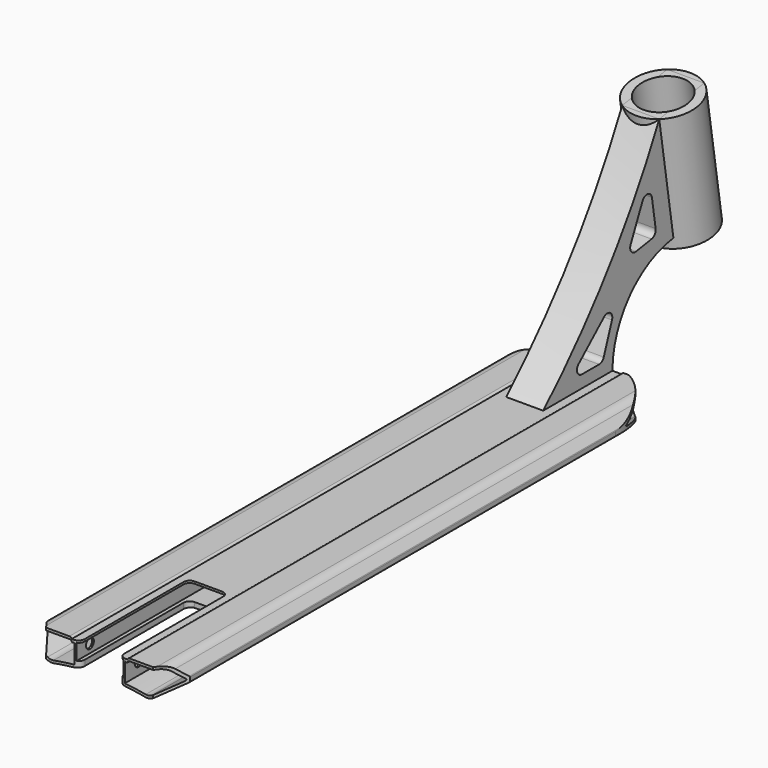
from build123d import *

# Parameters (mm, degrees)
F1_DEPTH       = 250
F2_W           = 38
F2_H           = 13
F3_DEPTH       = 250
F4_T1_DEPTH    = 509.3674969976
F5_R           = 9
F6_R           = 1
F8_DEPTH       = 500.001
F10_DEPTH      = 22.2193051812
F10_DEPTH_BACK = 1.301
F12_DEPTH      = 22.219305294
F12_DEPTH_BACK = 1.3010001
F13_T1_DEPTH   = 1.7268039449
F13_T6_DEPTH   = 34.5366784866
F13_S7_R       = 200
F13_T8_DEPTH   = 19
F13_T12_DEPTH  = 64.5366784866
F13_T18_DEPTH  = 31.7268039449
F13_S19_R      = 200
F13_T20_DEPTH  = 18
F13_T25_DEPTH  = 31.7268039449
F13_S26_R      = 200
F13_T27_DEPTH  = 18
F13_T32_DEPTH  = 64.5366784866
F13_T38_DEPTH  = 34.5366784866
F13_S39_R      = 200
F13_T40_DEPTH  = 19
F13_T41_DEPTH  = 61.7268039449
F15_DEPTH      = 15
F16_R          = 27.5
F17_DEPTH      = 100
F19_D          = 40
F21_D          = 8
F21_DEPTH      = 50
F21_TIP        = 2.4034424761
F23_DEPTH      = 42.5010001
F23_DEPTH_BACK = 72.5010001
F24_R          = 5


# Not quite as in the source:
# - a fillet or chamfer that OpenCascade refuses, or shapes differently, is made with other operations: its cross-section is extruded or revolved along the edge and cut away or added


with BuildPart() as f1:
    # F0 (on Front) → F1 (new body, symmetric)
    with BuildSketch(Plane.XZ):
        with BuildLine():
            Line((22.5, 0), (0, 0))
            Line((0, 0), (-22.5, 0))
            Line((-22.5, 0), (-22.5, 1.3))
            Line((-22.5, 1.3), (-49.1090036882, 1.3))
            Line((-49.1090036882, 1.3), (-57.5, -8.7))
            Line((-57.5, -8.7), (-57.5, -12.7))
            Line((-57.5, -12.7), (-40.1794919243, -22.7))
            ThreePointArc((-40.1794919243, -22.7), (0, -18.6224551416), (40.1794919243, -22.7))
            Line((40.1794919243, -22.7), (57.5, -12.7))
            Line((57.5, -12.7), (57.5, -8.7))
            Line((57.5, -8.7), (49.1090036882, 1.3))
            Line((49.1090036882, 1.3), (22.5, 1.3))
            Line((22.5, 1.3), (22.5, 0))
        make_face()
    extrude(amount=F1_DEPTH, both=True)

    # F2 (on Front) → F3 (cut, symmetric)
    with BuildSketch(Plane.XZ):
        with Locations((0, -8.2268039449)):
            Rectangle(F2_W, F2_H)
    extrude(amount=F3_DEPTH, both=True, mode=Mode.SUBTRACT)

    # F4: fillet of radius 2 on 2 edges, made by hand

    # F4_s2 → F4_t1 (cut)
    with BuildSketch(Plane.XZ.offset(-254.6837484988)):
        with BuildLine():
            ThreePointArc((24.3734993995, 1.3), (23.2333239744, 0.9431676725), (22.5, 0))
            Line((22.5, 0), (22.5, 1.3))
            Line((22.5, 1.3), (24.3734993995, 1.3))
        make_face()
        with BuildLine():
            ThreePointArc((-24.3734993995, 1.3), (-23.2333239744, 0.9431676725), (-22.5, 0))
            Line((-22.5, 0), (-22.5, 1.3))
            Line((-22.5, 1.3), (-24.3734993995, 1.3))
        make_face()
    extrude(amount=F4_T1_DEPTH, mode=Mode.SUBTRACT)

    # F5
    f5_edges = [f1.edges().sort_by_distance(p)[0] for p in [
        (-49.109004, 0, 1.3),
        (49.109004, 0, 1.3),
        (40.179492, 0, -22.7),
        (-40.179492, 0, -22.7),
    ]]
    fillet(f5_edges, radius=F5_R)

    # F6
    f6_edges = [f1.edges().sort_by_distance(p)[0] for p in [
        (-57.5, 0, -8.7),
        (-57.5, 0, -12.7),
        (57.5, 0, -8.7),
        (57.5, 0, -12.7),
    ]]
    fillet(f6_edges, radius=F6_R)

    # F7 (on face) → F8 (cut, through all)
    with BuildSketch(Plane.XZ.offset(250)):
        with BuildLine():
            ThreePointArc((-37.3093701274, -20.0978700124), (-28.8874083403, -18.698675567), (-20.4138456833, -17.6566000706))
            Line((-20.4138456833, -17.6566000706), (-20.4138456833, -2.3003034743))
            Line((-20.4138456833, -2.3003034743), (-22.4138456833, -2.3003034743))
            ThreePointArc((-22.4138456833, -2.3003034743), (-23.1084683824, -1.1509046105), (-24.3734993995, -0.7))
            Line((-24.3734993995, -0.7), (-44.9122347648, -0.7))
            ThreePointArc((-44.9122347648, -0.7), (-47.870562597, -1.3558454907), (-50.2745458667, -3.2004867322))
            Line((-50.2745458667, -3.2004867322), (-55.9308095341, -9.9413592785))
            ThreePointArc((-55.9308095341, -9.9413592785), (-56.149572844, -10.7577950659), (-55.664765091, -11.450172292))
            Line((-55.664765091, -11.450172292), (-42.1022690923, -19.2804830077))
            ThreePointArc((-42.1022690923, -19.2804830077), (-39.7790673433, -20.1186780608), (-37.3093701274, -20.0978700124))
        make_face()
        with BuildLine():
            Line((22.4138456833, -2.3003034743), (20.4138456833, -2.3003034743))
            Line((20.4138456833, -2.3003034743), (20.4138456833, -17.6566000706))
            ThreePointArc((20.4138456833, -17.6566000706), (28.8874083403, -18.698675567), (37.3093701274, -20.0978700124))
            ThreePointArc((37.3093701274, -20.0978700124), (39.7790673433, -20.1186780608), (42.1022690923, -19.2804830077))
            Line((42.1022690923, -19.2804830077), (55.664765091, -11.450172292))
            ThreePointArc((55.664765091, -11.450172292), (56.149572844, -10.7577950659), (55.9308095341, -9.9413592785))
            Line((55.9308095341, -9.9413592785), (50.2745458667, -3.2004867322))
            ThreePointArc((50.2745458667, -3.2004867322), (47.870562597, -1.3558454907), (44.9122347648, -0.7))
            Line((44.9122347648, -0.7), (24.3734993995, -0.7))
            ThreePointArc((24.3734993995, -0.7), (23.1084683824, -1.1509046105), (22.4138456833, -2.3003034743))
        make_face()
    extrude(amount=-F8_DEPTH, mode=Mode.SUBTRACT)

    # F9 (on Top) → F10 (cut, two sides)
    with BuildSketch(Plane.XY) as f10_sk:
        with BuildLine():
            ThreePointArc((-57.5, 200), (0, 257.5), (57.5, 200))
            Line((57.5, 200), (57.5, 280))
            Line((57.5, 280), (-57.5, 280))
            Line((-57.5, 280), (-57.5, 200))
        make_face()
    extrude(amount=-F10_DEPTH, mode=Mode.SUBTRACT)
    extrude(f10_sk.sketch, amount=F10_DEPTH_BACK, mode=Mode.SUBTRACT)

    # F11 (on Top) → F12 (cut, two sides)
    with BuildSketch(Plane.XY) as f12_sk:
        Polygon((16, -140), (-16, -140), (-16, -250), (-43.2975540478, -250), (-68, -216), (-68, -346), (68, -346), (68, -216), (43.2975540478, -250), (16, -250), align=None)
    extrude(amount=-F12_DEPTH, mode=Mode.SUBTRACT)
    extrude(f12_sk.sketch, amount=F12_DEPTH_BACK, mode=Mode.SUBTRACT)

    # F13: fillet of radius 5 on 6 edges, made by hand

    # F13_s2 → F13_t1 (join)
    with BuildSketch(Plane.XY.offset(-1.7268039449)):
        with BuildLine():
            ThreePointArc((-11, -140), (-14.5355339059, -141.4644660941), (-16, -145))
            Line((-16, -145), (-16.1, -145))
            Line((-16.1, -145), (-16.1, -139.9))
            Line((-16.1, -139.9), (-11, -139.9))
            Line((-11, -139.9), (-11, -140))
        make_face()
        with BuildLine():
            ThreePointArc((16, -145), (14.5355339059, -141.4644660941), (11, -140))
            Line((11, -140), (11, -139.9))
            Line((11, -139.9), (16.1, -139.9))
            Line((16.1, -139.9), (16.1, -145))
            Line((16.1, -145), (16, -145))
        make_face()
    extrude(amount=F13_T1_DEPTH)


with BuildPart() as f13_tool4:
    # F13_s5 → F13_t6 (new body)
    with BuildSketch(Plane.XY.offset(-49.2634824315)):
        with BuildLine():
            ThreePointArc((-16, -145), (-14.5355339059, -141.4644660941), (-11, -140))
            Line((-11, -140), (-11, -139.9))
            Line((-11, -139.9), (-16.1, -139.9))
            Line((-16.1, -139.9), (-16.1, -145))
            Line((-16.1, -145), (-16, -145))
        make_face()
    extrude(amount=F13_T6_DEPTH)

    # F13_s7 → F13_t8 (cut, symmetric)
    with BuildSketch(Plane.XZ.offset(142.4)):
        with Locations((0, -218.6224551416)):
            Circle(F13_S7_R)
    extrude(amount=F13_T8_DEPTH, both=True, mode=Mode.SUBTRACT)


with BuildPart() as f1_1:
    add(f1.part)

    # F13_t3: union F13_tool4
    add(f13_tool4.part)


with BuildPart() as f13_tool10:
    # F13_s11 → F13_t12 (new body)
    with BuildSketch(Plane.XY.offset(-49.2634824315)):
        with BuildLine():
            ThreePointArc((-16, -145), (-14.5355339059, -141.4644660941), (-11, -140))
            Line((-11, -140), (-11, -139.9))
            Line((-11, -139.9), (-16.1, -139.9))
            Line((-16.1, -139.9), (-16.1, -145))
            Line((-16.1, -145), (-16, -145))
        make_face()
    extrude(amount=F13_T12_DEPTH)

    split(bisect_by=Plane.XY.offset(-1.7268039449), keep=Keep.TOP)

    split(bisect_by=Plane.XY, keep=Keep.BOTTOM)


with BuildPart() as f1_2:
    add(f1_1.part)

    # F13_t9: union F13_tool10
    add(f13_tool10.part)


with BuildPart() as f13_tool16:
    # F13_s17 → F13_t18 (new body)
    with BuildSketch(Plane.XY.offset(-31.7268039449)):
        with BuildLine():
            ThreePointArc((-11, -140), (-14.5355339059, -141.4644660941), (-16, -145))
            Line((-16, -145), (-16.1, -145))
            Line((-16.1, -145), (-16.1, -139.9))
            Line((-16.1, -139.9), (-11, -139.9))
            Line((-11, -139.9), (-11, -140))
        make_face()
    extrude(amount=F13_T18_DEPTH)

    # F13_s19 → F13_t20 (cut, symmetric)
    with BuildSketch(Plane.XZ.offset(142.4)):
        with Locations((0, -218.6224551416)):
            Circle(F13_S19_R)
    extrude(amount=F13_T20_DEPTH, both=True, mode=Mode.SUBTRACT)

    split(bisect_by=Plane.XY.offset(-14.7268039449), keep=Keep.BOTTOM)


with BuildPart() as f1_3:
    add(f1_2.part)

    # F13_t15: union F13_tool16
    add(f13_tool16.part)


with BuildPart() as f13_tool23:
    # F13_s24 → F13_t25 (new body)
    with BuildSketch(Plane.XY):
        with BuildLine():
            ThreePointArc((16, -145), (14.5355339059, -141.4644660941), (11, -140))
            Line((11, -140), (11, -139.9))
            Line((11, -139.9), (16.1, -139.9))
            Line((16.1, -139.9), (16.1, -145))
            Line((16.1, -145), (16, -145))
        make_face()
    extrude(amount=-F13_T25_DEPTH)

    # F13_s26 → F13_t27 (cut, symmetric)
    with BuildSketch(Plane.XZ.offset(142.4)):
        with Locations((0, -218.6224551416)):
            Circle(F13_S26_R)
    extrude(amount=F13_T27_DEPTH, both=True, mode=Mode.SUBTRACT)

    split(bisect_by=Plane.XY.offset(-14.7268039449), keep=Keep.BOTTOM)


with BuildPart() as f1_4:
    add(f1_3.part)

    # F13_t22: union F13_tool23
    add(f13_tool23.part)


with BuildPart() as f13_tool30:
    # F13_s31 → F13_t32 (new body)
    with BuildSketch(Plane.XY.offset(15.2731960551)):
        with BuildLine():
            ThreePointArc((16, -145), (14.5355339059, -141.4644660941), (11, -140))
            Line((11, -140), (11, -139.9))
            Line((11, -139.9), (16.1, -139.9))
            Line((16.1, -139.9), (16.1, -145))
            Line((16.1, -145), (16, -145))
        make_face()
    extrude(amount=-F13_T32_DEPTH)

    split(bisect_by=Plane.XY.offset(-1.7268039449), keep=Keep.TOP)

    split(bisect_by=Plane.XY, keep=Keep.BOTTOM)


with BuildPart() as f1_5:
    add(f1_4.part)

    # F13_t29: union F13_tool30
    add(f13_tool30.part)


with BuildPart() as f13_tool36:
    # F13_s37 → F13_t38 (new body)
    with BuildSketch(Plane.XY.offset(-14.7268039449)):
        with BuildLine():
            ThreePointArc((16, -145), (14.5355339059, -141.4644660941), (11, -140))
            Line((11, -140), (11, -139.9))
            Line((11, -139.9), (16.1, -139.9))
            Line((16.1, -139.9), (16.1, -145))
            Line((16.1, -145), (16, -145))
        make_face()
    extrude(amount=-F13_T38_DEPTH)

    # F13_s39 → F13_t40 (cut, symmetric)
    with BuildSketch(Plane.XZ.offset(142.4)):
        with Locations((0, -218.6224551416)):
            Circle(F13_S39_R)
    extrude(amount=F13_T40_DEPTH, both=True, mode=Mode.SUBTRACT)


with BuildPart() as f1_6:
    add(f1_5.part)

    # F13_t35: union F13_tool36
    add(f13_tool36.part)

    # F13_s42 → F13_t41 (cut)
    with BuildSketch(Plane.XY.offset(-31.7268039449)):
        with BuildLine():
            ThreePointArc((-21, -250), (-17.4644660941, -248.5355339059), (-16, -245))
            Line((-16, -245), (-15.9, -245))
            Line((-15.9, -245), (-15.9, -250.1))
            Line((-15.9, -250.1), (-21, -250.1))
            Line((-21, -250.1), (-21, -250))
        make_face()
        with BuildLine():
            ThreePointArc((21, -250), (17.4644660941, -248.5355339059), (16, -245))
            Line((16, -245), (15.9, -245))
            Line((15.9, -245), (15.9, -250.1))
            Line((15.9, -250.1), (21, -250.1))
            Line((21, -250.1), (21, -250))
        make_face()
    extrude(amount=F13_T41_DEPTH, mode=Mode.SUBTRACT)

    # F14 (on Right) → F15 (join, symmetric)
    with BuildSketch(Plane.YZ):
        with BuildLine():
            Line((180, 0), (250, 0))
            ThreePointArc((250, 0), (267.6550746197, 46.4758946867), (311.7145367693, 69.5079211245))
            Line((311.7145367693, 69.5079211245), (313.0254460068, 61.2311659405))
            Line((313.0254460068, 61.2311659405), (358.4591096742, 68.4271513323))
            Line((358.4591096742, 68.4271513323), (342.8156631702, 167.1959853919))
            Line((342.8156631702, 167.1959853919), (297.3819995028, 160))
            ThreePointArc((297.3819995028, 160), (245.9666940414, 74.662277853), (180, 0))
        make_face()
    extrude(amount=F15_DEPTH, both=True)

    # F16 (on face) → F17 (join, through all)
    with BuildSketch(Plane(origin=(0, -17.4439040266, 110.1364754698), x_dir=(1, 0, 0), z_dir=(0, -0.156434465, 0.9876883406))):
        with Locations((0, 341.7502480182)):
            Circle(F16_R)
    extrude(amount=-F17_DEPTH)

    # F19 (through all)
    with Locations(Plane(origin=(0, -17.4439040266, 110.1364754698), x_dir=(1, 0, 0), z_dir=(0, -0.156434465, 0.9876883406))):
        with Locations((0, 341.7502480182)):
            Hole(F19_D / 2)

    # F21 (one way)
    with BuildSketch(Plane.YZ.offset(20.4138456833)):
        with Locations((-236, -7.7170047426)):
            Circle(F21_D / 2)
    extrude(amount=-F21_DEPTH, mode=Mode.SUBTRACT)
    with Locations(Plane.YZ.offset(20.4138456833)):
        with Locations((-236, -7.7170047426)):
            with Locations((0, 0, -(F21_DEPTH + F21_TIP / 2))):  # 118° drill point
                Cone(0, F21_D / 2, F21_TIP, mode=Mode.SUBTRACT)

    # F22 (on face) → F23 (cut, two sides)
    with BuildSketch(Plane.YZ.offset(15)) as f23_sk:
        Polygon((240, 10), (256.378660542, 55), (206, 10), align=None)
        Polygon((287.3447062809, 123.5418922598), (264.4720060955, 73.7903590501), (294.4720060955, 78.5418922598), align=None)
    extrude(amount=F23_DEPTH, mode=Mode.SUBTRACT)
    extrude(f23_sk.sketch, amount=-F23_DEPTH_BACK, mode=Mode.SUBTRACT)

    # F24
    f24_edges = [f1_6.edges().sort_by_distance(p)[0] for p in [
        (0, 294.472006, 78.541892),
        (0, 240, 10),
        (0, 256.378661, 55),
        (0, 287.344706, 123.541892),
        (0, 206, 10),
        (0, 264.472006, 73.790359),
    ]]
    fillet(f24_edges, radius=F24_R)


solid = f1_6.part
